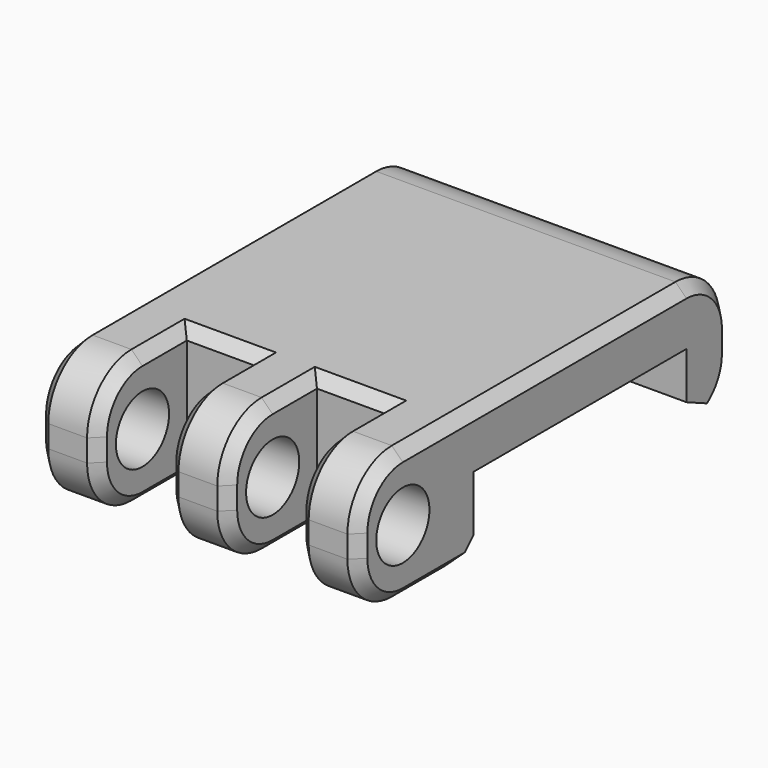
from build123d import *

# Parameters (mm, degrees)
F0_W        = 14.5
F0_H        = 21
F1_DEPTH    = 3
F2_R        = 1.5
F3_DEPTH    = 25
F4_R        = 2.5
F5_W        = 3.125
F5_H        = 5
F6_DEPTH    = 12.5
F7_W        = 14.5
F7_H        = 12
F8_DEPTH    = 3.5
F9_T1_DEPTH = 19.6433659759
F9_T3_DEPTH = 23.5630770458
F10_SIZE    = 0.5


# Not quite as in the source:
# - a fillet or chamfer that OpenCascade refuses, or shapes differently, is made with other operations: its cross-section is extruded or revolved along the edge and cut away or added


with BuildPart() as f1:
    # F0 (on Top) → F1 (new body, symmetric)
    with BuildSketch(Plane.XY):
        Rectangle(F0_W, F0_H)
    extrude(amount=F1_DEPTH, both=True)

    # F2 (on Right) → F3 (cut, symmetric)
    with BuildSketch(Plane.YZ):
        with Locations((-8, 0)):
            Circle(F2_R)
    extrude(amount=F3_DEPTH, both=True, mode=Mode.SUBTRACT)

    # F4
    f4_edges = [f1.edges().sort_by_distance(p)[0] for p in [
        (0, -10.5, 3),
        (0, -10.5, -3),
        (0, 10.5, 3),
        (0, 10.5, -3),
    ]]
    fillet(f4_edges, radius=F4_R)

    # F5 (on Top) → F6 (cut, symmetric)
    with BuildSketch(Plane.XY):
        with Locations((-2.9375, -8)):
            Rectangle(F5_W, F5_H)
        with Locations((2.9375, -8)):
            Rectangle(F5_W, F5_H)
    extrude(amount=F6_DEPTH, both=True, mode=Mode.SUBTRACT)

    # F7 (on face) → F8 (cut)
    with BuildSketch(Plane(origin=(0, 0, -3), x_dir=(1, 0, 0), z_dir=(0, 0, -1))):
        with Locations((0, -2)):
            Rectangle(F7_W, F7_H)
    extrude(amount=-F8_DEPTH, mode=Mode.SUBTRACT)

    # F9: chamfer of 1 on 2 edges, made by hand

    # F9_s2 → F9_t1 (cut)
    with BuildSketch(Plane.YZ.offset(-9.821682988)):
        Polygon((-5, -3), (-4, -2), (-4, -3), align=None)
    extrude(amount=F9_T1_DEPTH, mode=Mode.SUBTRACT)

    # F9_s4 → F9_t3 (cut)
    with BuildSketch(Plane.YZ.offset(-11.7815385229)):
        with BuildLine():
            Line((9.6666666667, -2.3633899812), (8, -1.6180339887))
            Line((8, -1.6180339887), (8, -3))
            ThreePointArc((8, -3), (8.906095825, -2.8300193896), (9.6666666667, -2.3633899812))
        make_face()
    extrude(amount=F9_T3_DEPTH, mode=Mode.SUBTRACT)

    # F10
    f10_edges = [f1.edges().sort_by_distance(p)[0] for p in [
        (-7.25, 0, 3),
        (-4.5, -6.75, 3),
        (-1.375, -6.75, 3),
        (1.375, -6.75, 3),
        (4.5, -6.75, 3),
        (7.25, 0, 3),
        (2.9375, -5.5, 3),
        (-2.9375, -5.5, 3),
        (-7.25, 10.5, 0),
        (7.25, 10.5, 0),
        (-7.25, 9.767767, 2.267767),
        (-7.25, -9.767767, 2.267767),
        (-7.25, -10.5, 0),
        (-7.25, -9.767767, -2.267767),
        (-7.25, -6.5, -3),
        (-7.25, 10.282177, -1.520621),
        (7.25, 10.282177, -1.520621),
        (7.25, 9.767767, 2.267767),
        (7.25, -9.767767, -2.267767),
        (7.25, -10.5, 0),
        (7.25, -9.767767, 2.267767),
        (7.25, -6.5, -3),
        (-4.5, -9.767767, 2.267767),
        (-4.5, -10.5, 0),
        (-4.5, -9.767767, -2.267767),
        (4.5, -6.75, -3),
        (1.375, -6.75, -3),
        (-1.375, -6.75, -3),
        (-4.5, -6.75, -3),
        (4.5, -9.767767, -2.267767),
        (4.5, -10.5, 0),
        (4.5, -9.767767, 2.267767),
        (1.375, -9.767767, 2.267767),
        (1.375, -10.5, 0),
        (1.375, -9.767767, -2.267767),
        (-1.375, -9.767767, 2.267767),
        (-1.375, -10.5, 0),
        (-1.375, -9.767767, -2.267767),
    ]]
    chamfer(f10_edges, length=F10_SIZE)


solid = f1.part
